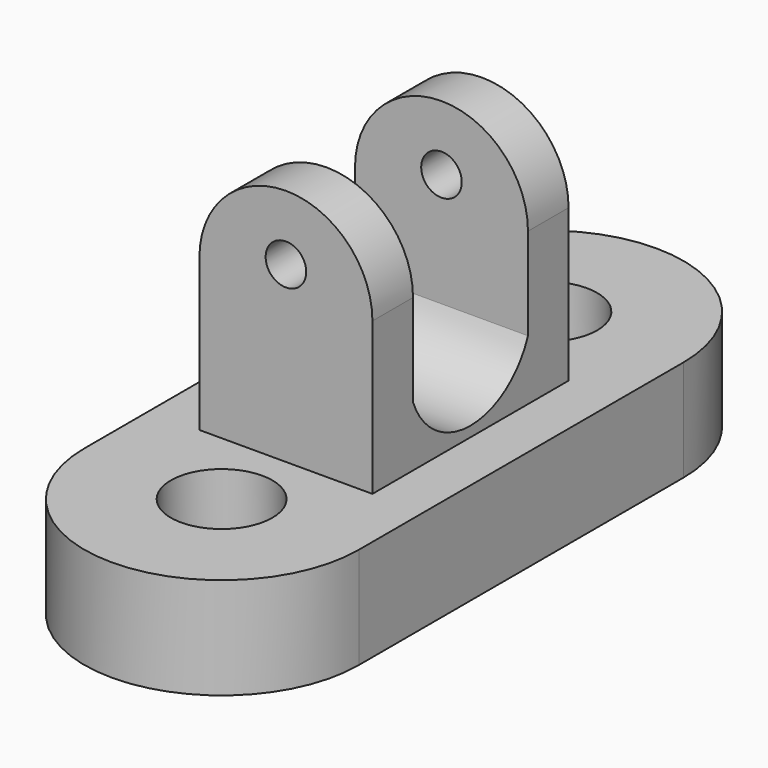
from build123d import *

# Parameters (mm, degrees)
F0_R     = 12.7
F1_DEPTH = 25.4
F3_DEPTH = 38.1
F5_DEPTH = 69.088
F7_R     = 5.08
F8_DEPTH = 12.7
F6_R     = 5.08
F9_DEPTH = 12.7


# Not quite as in the source:
# - a feature names something its author has since deleted; it is built from what else it names


with BuildPart() as f1:
    # F0 (on Top) → F1 (new body)
    with BuildSketch(Plane.XY):
        with BuildLine():
            Line((0, -55.3492553601), (0, 0))
            Line((0, 0), (0, 46.2507446399))
            ThreePointArc((0, 46.2507446399), (-34.3468652373, 80.5976098772), (-68.6937304746, 46.2507446399))
            Line((-68.6937304746, 46.2507446399), (-68.6937304746, -55.3492553601))
            ThreePointArc((-68.6937304746, -55.3492553601), (-34.3468652373, -89.6961205974), (0, -55.3492553601))
        make_face()
        with Locations((-34.3468652373, -55.3492553601)):
            Circle(F0_R, mode=Mode.SUBTRACT)
        with Locations((-34.3468652373, 46.2507446399)):
            Circle(F0_R, mode=Mode.SUBTRACT)
    extrude(amount=-F1_DEPTH)

    # F2 (on face) → F3 (join)
    with BuildSketch(Plane.XY):
        Polygon((-55.9937304746, 26.1313845437), (-55.9937304746, -4.5492553601), (-55.9937304746, -35.2298952639), (-12.7, -35.2298952639), (-12.7, -4.5492553601), (-12.7, 26.1313845437), align=None)
    extrude(amount=F3_DEPTH)

    # F4 (on face) → F5 (cut)
    with BuildSketch(Plane.YZ.offset(-12.7)):
        with BuildLine():
            Line((13.4313845437, 38.1), (-22.5298952639, 38.1))
            Line((-22.5298952639, 38.1), (-22.5298952639, 15.044502914))
            ThreePointArc((-22.5298952639, 15.044502914), (-4.5492553601, 2.5536219989), (13.4313845437, 15.044502914))
            Line((13.4313845437, 15.044502914), (13.4313845437, 38.1))
        make_face()
    extrude(amount=-F5_DEPTH, mode=Mode.SUBTRACT)

    # F7 (on face) → F8 (join)
    with BuildSketch(Plane(origin=(0, 26.1313845437, 0), x_dir=(-1, 0, 0), z_dir=(0, 1, 0))):
        with BuildLine():
            Line((12.7, 38.1), (55.9937304746, 38.1))
            ThreePointArc((55.9937304746, 38.1), (34.3468652373, 59.7468652373), (12.7, 38.1))
        make_face()
        with Locations((34.3468652373, 43.5117163093)):
            Circle(F7_R, mode=Mode.SUBTRACT)
    extrude(amount=-F8_DEPTH)

    # F6 (on face) → F9 (join)
    with BuildSketch(Plane.XZ.offset(35.2298952639)):
        with BuildLine():
            Line((-55.9937304746, 38.1), (-12.7, 38.1))
            ThreePointArc((-12.7, 38.1), (-34.3468652373, 59.7468652373), (-55.9937304746, 38.1))
        make_face()
        with Locations((-34.3468652373, 43.5117163093)):
            Circle(F6_R, mode=Mode.SUBTRACT)
    extrude(amount=-F9_DEPTH)


solid = f1.part
